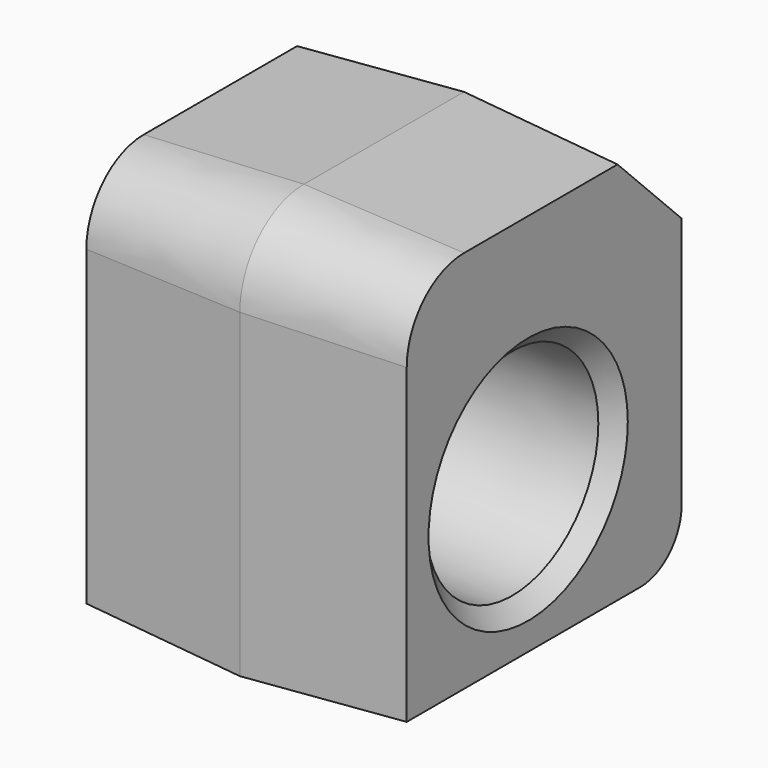
from build123d import *

# Parameters (mm, degrees)
F0_R     = 31.75
F1_DEPTH = 50.8
F1_TAPER = 3
F2_SIZE  = 25.4
F3_SIZE  = 5.08


with BuildPart() as f1:
    # F0 (on Right) → F1 (new body, symmetric)
    with BuildSketch(Plane.YZ):
        with BuildLine():
            Line((63.5, 76.2), (-25.4, 76.2))
            ThreePointArc((-25.4, 76.2), (-43.3605122421, 68.7605122421), (-50.8, 50.8))
            Line((-50.8, 50.8), (-50.8, -50.8))
            Line((-50.8, -50.8), (44.45, -50.8))
            ThreePointArc((44.45, -50.8), (57.9203841816, -45.2203841816), (63.5, -31.75))
            Line((63.5, -31.75), (63.5, 76.2))
        make_face()
        Circle(F0_R, mode=Mode.SUBTRACT)
    extrude(amount=F1_DEPTH, both=True, taper=F1_TAPER)

    # F2
    f2_edges = [f1.edges().sort_by_distance(p)[0] for p in [
        (25.4, 62.168842, 74.868842),
        (-25.4, 62.168842, 74.868842),
    ]]
    chamfer(f2_edges, length=F2_SIZE)

    # F3
    f3_edges = [f1.edges().sort_by_distance(p)[0] for p in [
        (50.8, -34.412315, 0),
    ]]
    chamfer(f3_edges, length=F3_SIZE)


solid = f1.part
